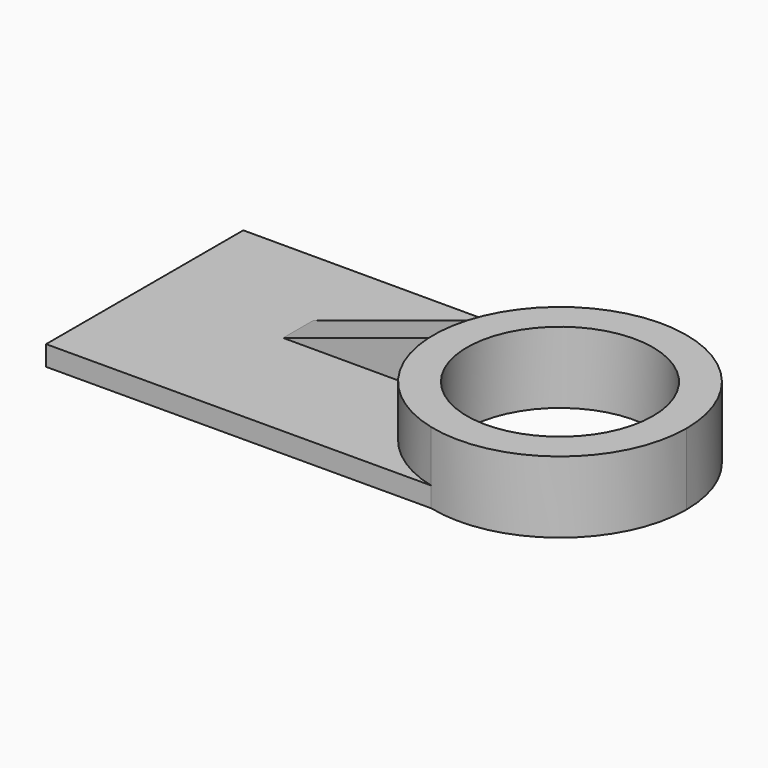
from build123d import *

# Parameters (mm, degrees)
F0_R     = 33.0333203714
F1_DEPTH = 25.4
F2_DEPTH = 7.112
F3_W     = 55.4855957025
F3_H     = 13.38801522
F4_DEPTH = 18.034
F7_DEPTH = 25.4


# Not quite as in the source:
# - a feature names something its author has since deleted; it is built from what else it names


with BuildPart() as f1:
    # F0 (on Top) → F1 (new body)
    with BuildSketch(Plane.XY):
        with BuildLine():
            ThreePointArc((-10.8790392065, -43.5892733327), (27.6552215769, -35.4057476022), (44.9263646842, 0))
            ThreePointArc((44.9263646842, 0), (27.6552215769, 35.4057476022), (-10.8790392065, 43.5892733327))
            ThreePointArc((-10.8790392065, 43.5892733327), (-44.9263646842, 0), (-10.8790392065, -43.5892733327))
        make_face()
        Circle(F0_R, mode=Mode.SUBTRACT)
    extrude(amount=F1_DEPTH)

    # F0 (on Top) → F2 (join)
    with BuildSketch(Plane.XY):
        with BuildLine():
            ThreePointArc((-10.8790392065, -43.5892733327), (27.6552215769, -35.4057476022), (44.9263646842, 0))
            ThreePointArc((44.9263646842, 0), (27.6552215769, 35.4057476022), (-10.8790392065, 43.5892733327))
            ThreePointArc((-10.8790392065, 43.5892733327), (-44.9263646842, 0), (-10.8790392065, -43.5892733327))
        make_face()
        Circle(F0_R, mode=Mode.SUBTRACT)
        with BuildLine():
            ThreePointArc((-10.8790392065, -43.5892733327), (-44.9263646842, 0), (-10.8790392065, 43.5892733327))
            Line((-10.8790392065, 43.5892733327), (-147.3678201437, 43.5892733327))
            Line((-147.3678201437, 43.5892733327), (-147.3678201437, -43.9813993871))
            Line((-147.3678201437, -43.9813993871), (-10.8790392065, -43.5892733327))
        make_face()
    extrude(amount=F2_DEPTH)

    # F3 (on face) → F4 (join)
    with BuildSketch(Plane.XY.offset(7.112)):
        with Locations((-70.6279851798, 6.69400761)):
            Rectangle(F3_W, F3_H)
    extrude(amount=F4_DEPTH)

    # F5 (on face) → F7 (cut)
    with BuildSketch(Plane(origin=(0, 13.38801522, 0), x_dir=(-1, 0, 0), z_dir=(0, 1, 0))):
        Polygon((42.8851873285, 25.146), (98.370783031, 7.112), (98.370783031, 25.146), align=None)
    extrude(amount=-F7_DEPTH, mode=Mode.SUBTRACT)


solid = f1.part
